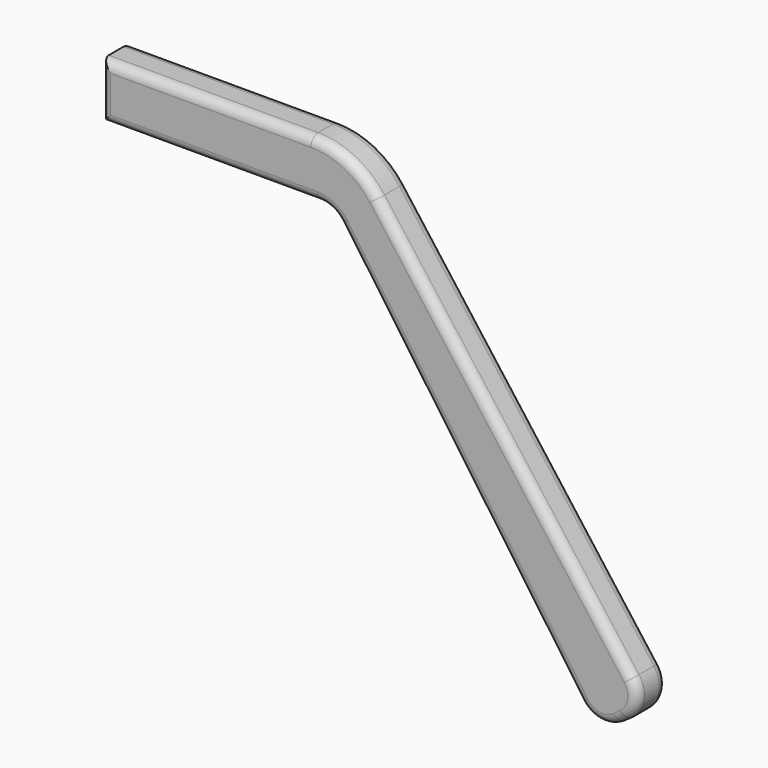
from build123d import *

# Parameters (mm, degrees)
F1_DEPTH = 2
F2_R     = 3
F3_R     = 9
F4_W     = 2
F4_H     = 5
F5_DEPTH = 10
F6_R     = 0.99999


# Not quite as in the source:
# - a fillet or chamfer is up to 0.001 mm smaller than in the source, because OpenCascade refuses the exact size


with BuildPart() as f1:
    # F0 (on Front) → F1 (new body, symmetric)
    with BuildSketch(Plane.XZ):
        Polygon((27.2452607751, 0), (0, 0), (0, -6), (25, -6), (53.6788218176, -46.9576022144), (59.4128861276, -42.94256716), align=None)
    extrude(amount=F1_DEPTH, both=True)

    # F2
    f2_edges = [f1.edges().sort_by_distance(p)[0] for p in [
        (25, 0, -6),
        (53.678822, 0, -46.957602),
        (59.412886, 0, -42.942567),
    ]]
    fillet(f2_edges, radius=F2_R)

    # F3
    f3_edges = [f1.edges().sort_by_distance(p)[0] for p in [
        (27.245261, 0, 0),
    ]]
    fillet(f3_edges, radius=F3_R)

    # F4 (on face) → F5 (cut)
    with BuildSketch(Plane(origin=(0, 0, 0), x_dir=(0, -1, 0), z_dir=(-1, 0, 0))):
        with Locations((0, -3)):
            Rectangle(F4_W, F4_H)
    extrude(amount=-F5_DEPTH, mode=Mode.SUBTRACT)

    # F6 (radius 1 in the source; OpenCascade refuses exactly that, so slightly less here)
    f6_edges = [f1.edges().sort_by_distance(p)[0] for p in [
        (43.750416, -2, -22.03376),
        (26.769245, -2, -0.951335),
        (58.117041, -2, -42.735428),
        (11.370982, -2, 0),
        (56.505829, -2, -44.978111),
        (0, -2, -3),
        (53.894604, -2, -45.73384),
        (11.719149, -2, -6),
        (38.926924, -2, -25.889708),
        (24.823545, -2, -6.338968),
        (43.750416, 2, -22.03376),
        (26.769245, 2, -0.951335),
        (58.117041, 2, -42.735428),
        (11.370982, 2, 0),
        (56.505829, 2, -44.978111),
        (0, 2, -3),
        (53.894604, 2, -45.73384),
        (11.719149, 2, -6),
        (38.926924, 2, -25.889708),
        (24.823545, 2, -6.338968),
    ]]
    fillet(f6_edges, radius=F6_R)


solid = f1.part
